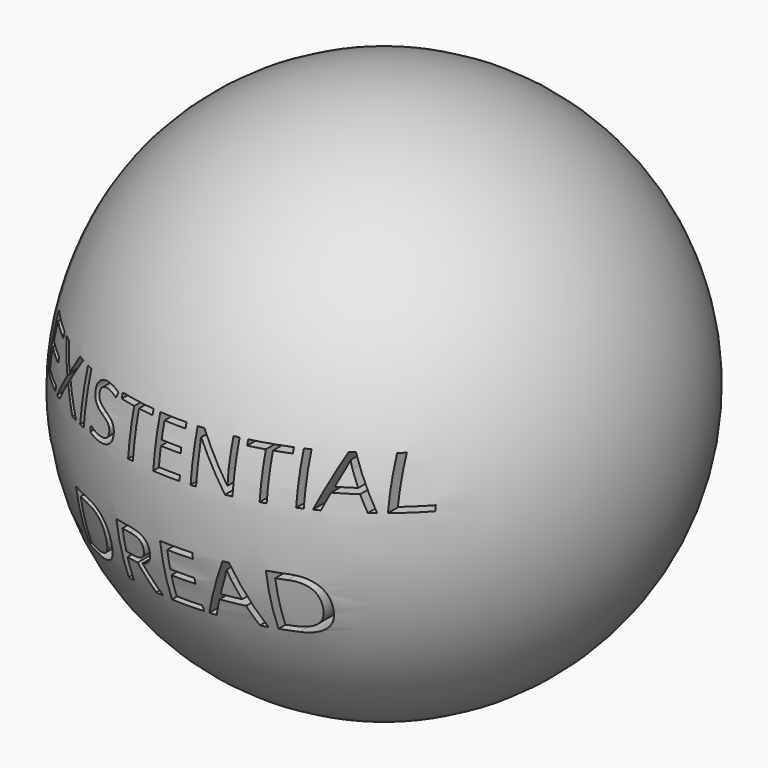
from build123d import *

# Parameters (mm, degrees)
F3_START        = 12.7
F2_TEXT_SIZE    = 6.5128205128
F2_TEXT_SIZE_2  = 7.7701830696
F3_DEPTH        = 12.7
F5_R            = 25.4
F6_DEPTH        = 3.175
F7_R            = 12.7
F9_START        = -23.8125
F8_R            = 25.4
F9_DEPTH        = 1.5875
F10_R           = 12.7
F11_TEXT_SIZE   = 4.1022880215
F11_TEXT_SIZE_2 = 1.9646137484
F12_DEPTH       = 3.175


# Not quite as in the source:
# - Text() gives the source's letters only with a copy of the font that has no kerning and outlines rounded to 1/6400 em; it was checked with that copy


with BuildPart() as f1:
    # F0 (on Front) → F1 (revolve)
    with BuildSketch(Plane.XZ):
        with BuildLine():
            Line((0, -25.4), (0, 25.4))
            ThreePointArc((0, 25.4), (-25.4, 0), (0, -25.4))
        make_face()
    revolve(axis=Axis((0, 0, 0), (0, 0, -1)))

    # F2 (on Front) → F3 (cut)
    with BuildSketch(Plane.XZ.offset(F3_START)):
        with Locations((-19.05, 2.232914)):
            Text('EXISTENTIAL', F2_TEXT_SIZE, font='Open Sans', text_align=(TextAlign.LEFT, TextAlign.BOTTOM))
        with Locations((-12.7, -9.1059122144)):
            Text('DREAD', F2_TEXT_SIZE_2, font='Open Sans', text_align=(TextAlign.LEFT, TextAlign.BOTTOM))
    extrude(amount=F3_DEPTH, mode=Mode.SUBTRACT)

    # F5 (on offset) → F6 (cut)
    with BuildSketch(Plane.YZ.offset(-25.4)):
        Circle(F5_R)
    extrude(amount=F6_DEPTH, mode=Mode.SUBTRACT)

    # F7
    f7_edges = [f1.edges().sort_by_distance(p)[0] for p in [
        (-22.225, 12.296722, 0),
        (-22.225, -12.296722, 0),
    ]]
    fillet(f7_edges, radius=F7_R)

    # F8 (on Front) → F9 (cut)
    with BuildSketch(Plane.XZ.offset(F9_START)):
        Circle(F8_R)
    extrude(amount=-F9_DEPTH, mode=Mode.SUBTRACT)

    # F10
    f10_edges = [f1.edges().sort_by_distance(p)[0] for p in [
        (0, 23.8125, 8.838826),
    ]]
    fillet(f10_edges, radius=F10_R)

    # F11 (on face) → F12 (cut)
    with BuildSketch(Plane(origin=(0, 23.8125, 0), x_dir=(-1, 0, 0), z_dir=(0, 1, 0))):
        with Locations((-4.7625, 0.635)):
            Text('Shen', F11_TEXT_SIZE, font='Open Sans', text_align=(TextAlign.LEFT, TextAlign.BOTTOM))
        with Locations((-4.7625, -2.0495218989)):
            Text('Blue Chair', F11_TEXT_SIZE_2, font='Open Sans', text_align=(TextAlign.LEFT, TextAlign.BOTTOM))
    extrude(amount=-F12_DEPTH, mode=Mode.SUBTRACT)


solid = f1.part
